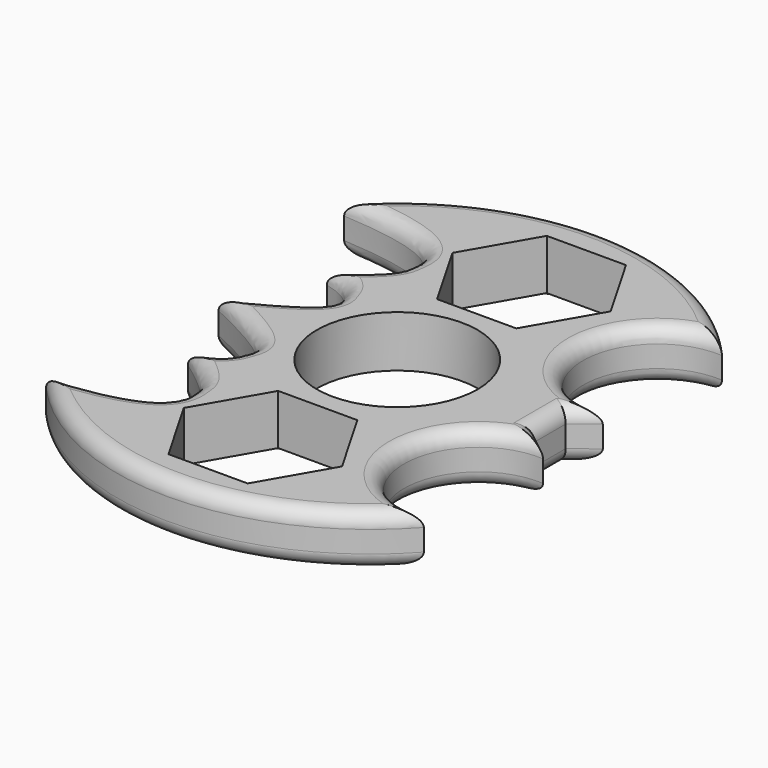
from build123d import *

# Parameters (mm, degrees)
F0_R     = 10.9474
F1_DEPTH = 7.0104
F2_R     = 2.032
F3_R     = 11.2199177984
F3_R_2   = 10.9474
F3_R_3   = 11.2453296403
F3_R_4   = 10.922
F4_DEPTH = 6.858


# Not quite as in the source:
# - a feature names something its author has since deleted; it is built from what else it names


with BuildPart() as f1:
    # F0 (on Top) → F1 (new body)
    with BuildSketch(Plane.XY):
        with BuildLine():
            Line((20.810874179, -2.6461168255), (20.810874179, 0))
            Line((20.810874179, 0), (20.810874179, 2.6461168255))
            Line((20.810874179, 2.6461168255), (23.9177607, 5.0893152782))
            ThreePointArc((23.9177607, 5.0893152782), (13.1070644437, 15.2284569767), (23.9177607, 25.3675986752))
            ThreePointArc((23.9177607, 25.3675986752), (-1.8005329696, 36.8526905137), (-27.5188266391, 25.3675986752))
            add(Edge.make_bspline(
                [(-27.5188266391, 25.3675986752), (-12.560030152, 24.4426897076), (-13.0047335039, 17.9656622926), (-13.3763186119, 15.952395202), (-19.0493152676, 11.8175025732)],
                knots=[0, 0, 0, 0, 0.5718814963, 1, 1, 1, 1], degree=3))
            add(Edge.make_bspline(
                [(-19.0493152676, 11.8175025732), (-15.1437984504, 10.7986718495), (-14.1130191842, 7.3272586693), (-13.1873289518, 5.3002074967), (-24.3299100548, 0)],
                knots=[0, 0, 0, 0, 0.403504276, 1, 1, 1, 1], degree=3))
            add(Edge.make_bspline(
                [(-19.0493152676, -11.8175025732), (-15.1437984504, -10.7986718495), (-14.1130191842, -7.3272586693), (-13.1873289518, -5.3002074967), (-24.3299100548, 0)],
                knots=[0, 0, 0, 0, 0.403504276, 1, 1, 1, 1], degree=3))
            add(Edge.make_bspline(
                [(-27.5188266391, -25.3675986752), (-12.560030152, -24.4426897076), (-13.0047335039, -17.9656622926), (-13.3763186119, -15.952395202), (-19.0493152676, -11.8175025732)],
                knots=[0, 0, 0, 0, 0.5718814963, 1, 1, 1, 1], degree=3))
            ThreePointArc((-27.5188266391, -25.3675986752), (-1.8005329696, -36.8526905137), (23.9177607, -25.3675986752))
            ThreePointArc((23.9177607, -25.3675986752), (13.1070644437, -15.2284569767), (23.9177607, -5.0893152782))
            Line((23.9177607, -5.0893152782), (20.810874179, -2.6461168255))
        make_face()
        with BuildLine():
            ThreePointArc((-4.0767593454, -12.7), (0, -11.9126), (4.0767593454, -12.7))
            ThreePointArc((4.0767593454, -12.7), (9.0685026884, -16.7274780268), (10.9474, -22.86))
            ThreePointArc((10.9474, -22.86), (-6.1325219732, -31.9285026884), (-4.0767593454, -12.7))
        make_face(mode=Mode.SUBTRACT)
        Circle(F0_R, mode=Mode.SUBTRACT)
        with BuildLine():
            ThreePointArc((10.922, 22.86), (9.0295634517, 16.715321988), (4.0080523949, 12.7))
            ThreePointArc((4.0080523949, 12.7), (0, 11.938), (-4.0080523949, 12.7))
            ThreePointArc((-4.0080523949, 12.7), (-6.144678012, 31.8895634517), (10.922, 22.86))
        make_face(mode=Mode.SUBTRACT)
    extrude(amount=F1_DEPTH)

    # F2
    f2_edges = [f1.edges().sort_by_distance(p)[0] for p in [
        (-1.800533, 36.852691, 7.0104),
        (-1.800533, 36.852691, 0),
        (-1.800533, -36.852691, 0),
        (-1.800533, -36.852691, 7.0104),
        (13.107064, -15.228457, 7.0104),
        (13.107064, 15.228457, 7.0104),
        (13.107064, -15.228457, 0),
        (13.107064, 15.228457, 0),
        (20.810874, 0, 0),
        (20.810874, 0, 7.0104),
        (22.364317, 3.867716, 7.0104),
        (22.364317, 3.867716, 0),
        (22.364317, -3.867716, 7.0104),
        (22.364317, -3.867716, 0),
        (-14.449366, -22.32097, 7.0104),
        (-15.518864, -4.931925, 7.0104),
        (-15.518864, 4.931925, 7.0104),
        (-14.449366, 22.32097, 7.0104),
        (-14.449366, 22.32097, 0),
        (-15.518864, 4.931925, 0),
        (-15.518864, -4.931925, 0),
        (-14.449366, -22.32097, 0),
    ]]
    fillet(f2_edges, radius=F2_R)

    # F3 (on face) → F4 (join)
    with BuildSketch(Plane.XY.offset(7.0104)):
        with Locations((0, -22.86)):
            Circle(F3_R)
        with Locations((0, -22.86)):
            Circle(F3_R_2, mode=Mode.SUBTRACT)
        with Locations((0, 22.86)):
            Circle(F3_R_3)
        with Locations((0, 22.86)):
            Circle(F3_R_4, mode=Mode.SUBTRACT)
        with Locations((0, -22.86)):
            Circle(F3_R_2)
        Polygon((-10.7785521755, -22.86), (-5.3892760878, -13.5255), (5.3892760878, -13.5255), (10.7785521755, -22.86), (5.3892760878, -32.1945), (-5.3892760878, -32.1945), align=None, mode=Mode.SUBTRACT)
        with Locations((0, 22.86)):
            Circle(F3_R_4)
        Polygon((-10.7785521755, 22.86), (-5.3892760878, 32.1945), (5.3892760878, 32.1945), (10.7785521755, 22.86), (5.3892760878, 13.5255), (-5.3892760878, 13.5255), align=None, mode=Mode.SUBTRACT)
    extrude(amount=-F4_DEPTH)


solid = f1.part
